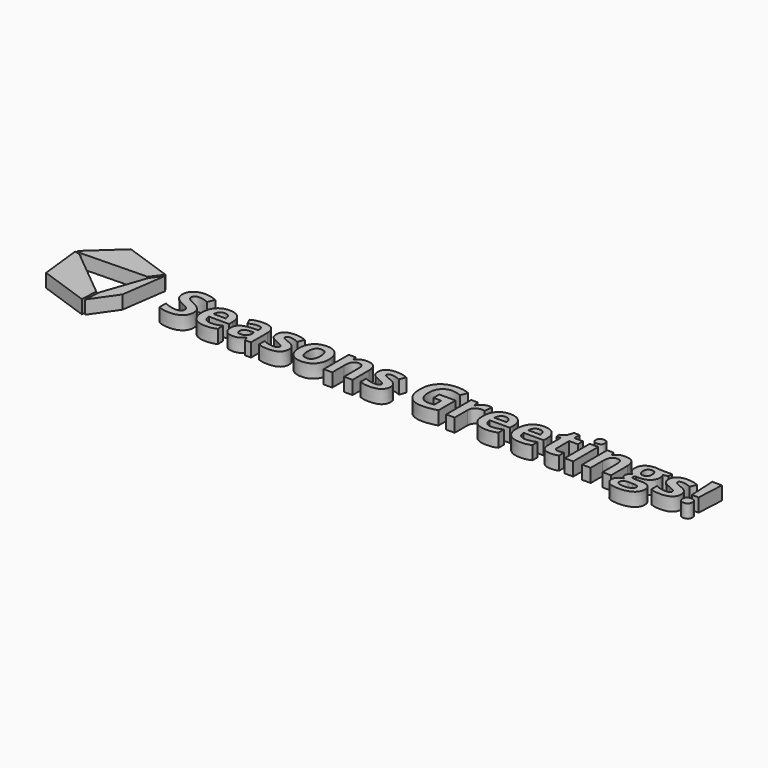
from build123d import *

# Parameters (mm, degrees)
F0_TEXT_SIZE = 8.5225381184
F1_DEPTH     = 2


# Not quite as in the source:
# - Text() gives the source's letters only with a copy of the font that has no kerning and outlines rounded to 1/6400 em; it was checked with that copy


with BuildPart() as f1:
    # F0 (on Top) → F1 (new body)
    with BuildSketch(Plane.XY):
        Polygon((-5.178323, 1.943723), (-5.999979, 2.202277), (-5.298557, -4.102247), (2.086005, -6.683141), (2.224498, -4.157713), align=None)
        Polygon((5.040174, -2.819294), (5.999978, 3.891408), (4.818655, 2.266873), (2.593812, -4.185446), (2.455319, -6.511575), align=None)
        Polygon((-5.10012, 2.262394), (4.560273, 2.488393), (5.833924, 4.195954), (-1.292256, 6.683141), (-5.86183, 2.488393), align=None)
        with Locations((10, -2.8960620963)):
            Text('Seasons Greetings!', F0_TEXT_SIZE, font='Open Sans', font_style=FontStyle.BOLD, text_align=(TextAlign.LEFT, TextAlign.BOTTOM))
    extrude(amount=F1_DEPTH)


solid = f1.part
